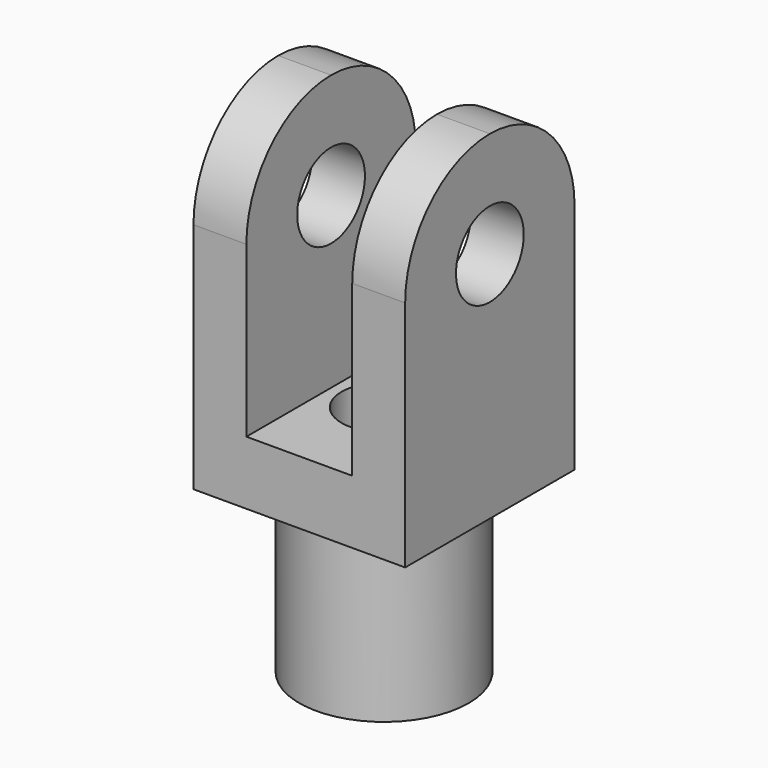
from build123d import *

# Parameters (mm, degrees)
F1_DEPTH = 50
F3_D     = 20
F4_R     = 20
F5_DEPTH = 40
F7_D     = 20
F8_R     = 24.99999


# Not quite as in the source:
# - a fillet or chamfer is up to 0.001 mm smaller than in the source, because OpenCascade refuses the exact size


with BuildPart() as f1:
    # F0 (on Front) → F1 (new body)
    with BuildSketch(Plane.XZ):
        Polygon((-25, 0), (0, 0), (25, 0), (25, 80), (12.5, 80), (12.5, 15), (0, 15), (-12.5, 15), (-12.5, 80), (-25, 80), align=None)
    extrude(amount=F1_DEPTH)

    # F3 (through all)
    with Locations(Plane(origin=(-25, 0, 0), x_dir=(0, -1, 0), z_dir=(-1, 0, 0))):
        with Locations((25, 55)):
            Hole(F3_D / 2)

    # F4 (on face) → F5 (join)
    with BuildSketch(Plane(origin=(0, 0, 0), x_dir=(1, 0, 0), z_dir=(0, 0, -1))):
        with Locations((0, 25)):
            Circle(F4_R)
    extrude(amount=F5_DEPTH)

    # F7 (through all)
    with Locations(Plane(origin=(0, 0, -40), x_dir=(1, 0, 0), z_dir=(0, 0, -1))):
        with Locations((0, 25)):
            Hole(F7_D / 2)

    # F8 (radius 25 in the source; OpenCascade refuses exactly that, so slightly less here)
    f8_edges = [f1.edges().sort_by_distance(p)[0] for p in [
        (18.75, -50, 80),
        (18.75, 0, 80),
        (-18.75, -50, 80),
        (-18.75, 0, 80),
    ]]
    fillet(f8_edges, radius=F8_R)


solid = f1.part
